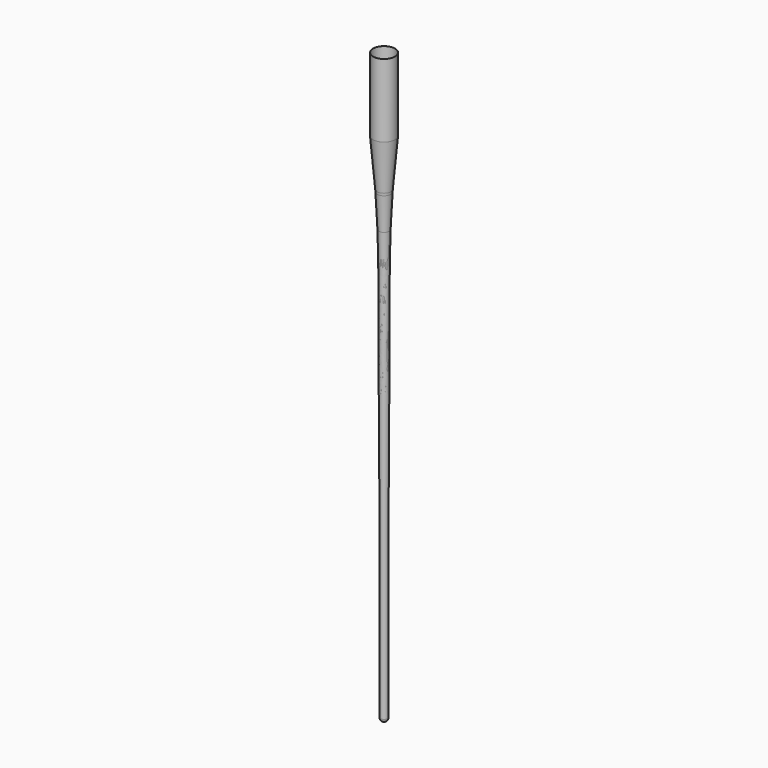
from build123d import *


# Not quite as in the source:
# - ends of sketch curves that miss each other by under 0.0002 mm in the source are joined
# - the dataset's text gives a spline's control points without its knots; the knots are read off the source's solid


with BuildPart() as f1:
    # F0 (on Front) → F1 (revolve)
    with BuildSketch(Plane.XZ):
        with BuildLine():
            Line((1.5, 80), (1.49, 80))
            Line((1.49, 80), (1.49, 70))
            add(Edge.make_bspline(
                [(1.49, 70), (1.1897983225, 66.8721229494), (0.5224322281, 59.9186671645), (0.6416749933, 44.4177535042), (0.4333089579, 29.6111831977), (0.4690584997, 10.9382819568), (0.49, 0)],
                knots=[0, 0, 0, 0, 0.1932096466, 0.4295164782, 0.6658200281, 1, 1, 1, 1], degree=3))
            ThreePointArc((0.49, 0), (0.3464823228, -0.3464823228), (0, -0.49))
            Line((0, -0.49), (0, -0.5))
            ThreePointArc((0, -0.5), (0.3538916697, -0.3532147875), (0.4999990837, 0.0009572555))
            add(Edge.make_bspline(
                [(1.4999086219, 69.9985691275), (1.4028137471, 68.9869131903), (1.2085847069, 66.9636288325), (0.9480089106, 63.8027077269), (0.7479566181, 60.3943974582), (0.6420287243, 56.5992185989), (0.6035813453, 52.5644646836), (0.6012019408, 49.1465540782), (0.6019932964, 46.4604972796), (0.5990362983, 43.838363027), (0.5818777012, 40.7020480392), (0.550270693, 36.9312953236), (0.5221685074, 33.601101934), (0.5032373155, 30.7148084657), (0.4920978701, 28.4075433872), (0.4841182848, 25.9599787242), (0.4771506194, 22.5315925844), (0.4746150972, 17.9696289095), (0.4789662342, 12.1639232621), (0.4882498116, 6.1375192021), (0.4960822008, 2.0463764302), (0.4999990837, 0.0009572555)],
                knots=[9.7906e-06, 9.7906e-06, 9.7906e-06, 9.7906e-06, 0.0625, 0.125, 0.1875, 0.25, 0.3125, 0.375, 0.40625, 0.4375, 0.5, 0.5625, 0.625, 0.65625, 0.6875, 0.71875, 0.75, 0.8125, 0.875, 0.9375, 0.9999904465, 0.9999904465, 0.9999904465, 0.9999904465], degree=3))
            Line((1.4999086219, 69.9985691275), (1.5, 70))
            Line((1.5, 70), (1.5, 80))
        make_face()
    revolve(axis=Axis((0, 0, 40), (0, 0, 1)))


solid = f1.part
